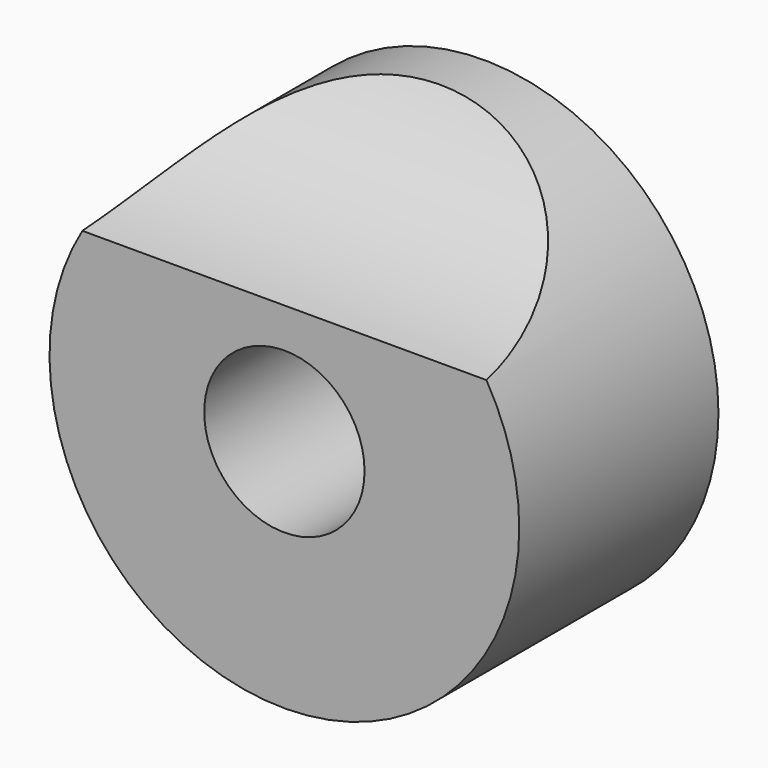
from build123d import *

# Parameters (mm, degrees)
F0_R     = 12.45
F0_R_2   = 4.25
F1_DEPTH = 13.2
F3_DEPTH = 12.5


with BuildPart() as f1:
    # F0 (on Front) → F1 (new body)
    with BuildSketch(Plane.XZ):
        Circle(F0_R)
        Circle(F0_R_2, mode=Mode.SUBTRACT)
    extrude(amount=F1_DEPTH)

    # F2 (on Right) → F3 (cut, symmetric)
    with BuildSketch(Plane.YZ):
        with BuildLine():
            Line((-2.87, 12.45), (-13.2, 12.45))
            Line((-13.2, 12.45), (-13.2, 6.35))
            ThreePointArc((-13.2, 6.35), (-7.4416487749, 8.3951937451), (-2.87, 12.45))
        make_face()
    extrude(amount=F3_DEPTH, both=True, mode=Mode.SUBTRACT)


solid = f1.part
